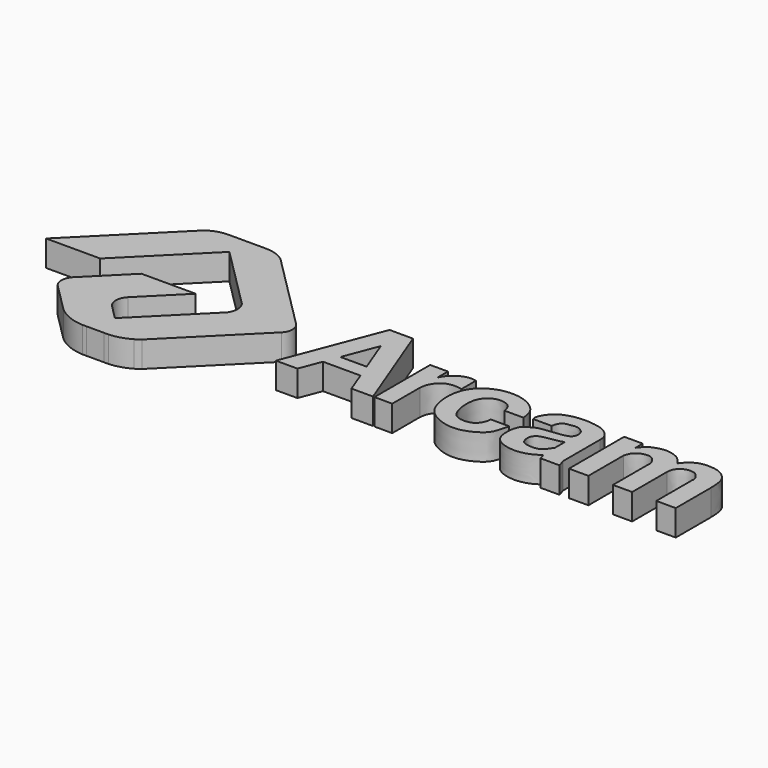
from build123d import *

# Parameters (mm, degrees)
F1_DEPTH = 2


# Not quite as in the source:
# - ends of sketch curves that miss each other by under 0.0002 mm in the source are joined


with BuildPart() as f1:
    # F0 (on Top) → F1 (new body)
    with BuildSketch(Plane.XY):
        with BuildLine():
            Line((-68.5442758233, 37.8376201657), (-75.2842758233, 31.0976201657))
            Line((-75.2842758233, 31.0976201657), (-71.1123458143, 31.0976201657))
            Line((-71.1123458143, 31.0976201657), (-65.5848875755, 36.6250784045))
            Line((-65.5848875755, 36.6250784045), (-64.6773347005, 37.5326312795))
            ThreePointArc((-64.6773347005, 37.5326312795), (-63.7017726464, 38.0238729513), (-62.6255051316, 37.8376259696))
            ThreePointArc((-62.6255051316, 37.8376259696), (-63.3349333998, 38.2093307968), (-64.1254993276, 38.3376213265))
            Line((-64.1254993276, 38.3376213265), (-67.0442758233, 38.3376201657))
            ThreePointArc((-67.0442758233, 38.3376201657), (-67.8348452384, 38.2093284108), (-68.5442758233, 37.8376201657))
        make_face()
        with BuildLine():
            Line((-64.6773347005, 37.5326312795), (-65.5848875755, 36.6250784045))
            Line((-65.5848875755, 36.6250784045), (-60.7645361178, 31.8047269468))
            ThreePointArc((-60.7645361178, 31.8047269468), (-60.5380345874, 31.0976201657), (-60.7645361178, 30.3905133845))
            Line((-60.7645361178, 30.3905133845), (-65.5722546007, 25.5827949015))
            Line((-65.5722546007, 25.5827949015), (-64.4237848444, 24.4343251452))
            ThreePointArc((-64.4237848444, 24.4343251452), (-63.7272467457, 24.0680817951), (-62.9458155435, 24.161166653))
            ThreePointArc((-62.9458155435, 24.161166653), (-62.7347896268, 24.2795555552), (-62.5487943481, 24.4343251452))
            Line((-62.5487943481, 24.4343251452), (-56.5926061088, 30.3905133845))
            ThreePointArc((-56.5926061088, 30.3905133845), (-56.29971289, 31.0976201657), (-56.5926061088, 31.8047269468))
            Line((-56.5926061088, 31.8047269468), (-62.6255051316, 37.8376259696))
            ThreePointArc((-62.6255051316, 37.8376259696), (-63.7017726464, 38.0238729513), (-64.6773347005, 37.5326312795))
        make_face()
        with BuildLine():
            Line((-64.4237848444, 24.4343251452), (-65.5722546007, 25.5827949015))
            Line((-65.5722546007, 25.5827949015), (-66.6552237276, 26.6657640284))
            ThreePointArc((-66.6552237276, 26.6657640284), (-66.9745179706, 27.4366085204), (-66.6552237276, 28.2074530124))
            Line((-66.6552237276, 28.2074530124), (-63.7650565743, 31.0976201657))
            Line((-63.7650565743, 31.0976201657), (-67.9369865833, 31.0976201657))
            Line((-67.9369865833, 31.0976201657), (-70.9051354279, 28.1294713211))
            ThreePointArc((-70.9051354279, 28.1294713211), (-71.1618860391, 27.4698706738), (-70.9545111372, 26.793121429))
            Line((-70.9545111372, 26.793121429), (-68.7112460172, 24.549856309))
            ThreePointArc((-68.7112460172, 24.549856309), (-67.7067925748, 23.9297700279), (-66.5533270991, 23.6788694294))
            Line((-66.5533270991, 23.6788694294), (-66.2402591376, 23.6788694294))
            Line((-66.2402591376, 23.6788694294), (-64.9042500639, 23.6788694294))
            Line((-64.9042500639, 23.6788694294), (-64.5486833954, 23.6788694294))
            ThreePointArc((-64.5486833954, 23.6788694294), (-63.7179930832, 23.8227872907), (-62.9458155435, 24.161166653))
            ThreePointArc((-62.9458155435, 24.161166653), (-63.7272467457, 24.0680817951), (-64.4237848444, 24.4343251452))
        make_face()
        with BuildLine():
            ThreePointArc((-64.9042500639, 23.6788694294), (-64.7264667296, 23.6743512397), (-64.5486833954, 23.6788694294))
            Line((-64.5486833954, 23.6788694294), (-64.9042500639, 23.6788694294))
        make_face()
        with BuildLine():
            ThreePointArc((-66.5533270991, 23.6788694294), (-66.3967931184, 23.6753672648), (-66.2402591376, 23.6788694294))
            Line((-66.2402591376, 23.6788694294), (-66.5533270991, 23.6788694294))
        make_face()
    extrude(amount=F1_DEPTH)


with BuildPart() as f1b:
    # F0 (on Top) → F1, piece 2 (new body)
    with BuildSketch(Plane.XY):
        Polygon((-51.7120547432, 34.7021047027), (-54.5506963793, 27.307190418), (-52.8916748268, 27.307190418), (-52.2540972099, 28.9681368956), (-49.3647159226, 28.9681368956), (-48.7271383057, 27.307190418), (-47.0681167532, 27.307190418), (-49.9067583893, 34.7021047027), align=None)
        Polygon((-49.8006260827, 30.103721687), (-51.8181870498, 30.103721687), (-50.8094065663, 32.7316846933), align=None, mode=Mode.SUBTRACT)
    extrude(amount=F1_DEPTH)


with BuildPart() as f1c:
    # F0 (on Top) → F1, piece 3 (new body)
    with BuildSketch(Plane.XY):
        with BuildLine():
            Line((-46.9542004939, 32.6685147129), (-46.9542004939, 27.3020714057))
            Line((-46.9542004939, 27.3020714057), (-45.5843665477, 27.3020714057))
            Line((-45.5843665477, 27.3020714057), (-45.5843665477, 29.9733391266))
            add(Edge.make_bspline(
                [(-43.5228206988, 31.4098937788), (-43.7790188564, 31.4438715653), (-44.2889116925, 31.5114951193), (-45.0377190249, 31.2578918185), (-45.509767693, 30.5488637582), (-45.5609753311, 30.153800628), (-45.5843665477, 29.9733391266)],
                knots=[0, 0, 0, 0, 0.257839139, 0.513158764, 0.777615035, 1, 1, 1, 1], degree=3))
            Line((-43.5228206988, 31.4098937788), (-43.5228206988, 32.7752627899))
            add(Edge.make_bspline(
                [(-45.5843665477, 31.6332013581), (-45.5308791384, 31.7621508466), (-45.4091654003, 32.0555829737), (-44.8749149339, 32.5566936661), (-44.3047762851, 32.8102137143), (-43.8681395106, 32.8598250997), (-43.634032553, 32.8024965546), (-43.5228206988, 32.7752627899)],
                knots=[0, 0, 0, 0, 0.1877342824, 0.4272003744, 0.6508029702, 0.8341149295, 1, 1, 1, 1], degree=3))
            Line((-45.5843665477, 31.6332013581), (-45.5843665477, 32.6685147129))
            Line((-45.5843665477, 32.6685147129), (-46.9542004939, 32.6685147129))
        make_face()
    extrude(amount=F1_DEPTH)


with BuildPart() as f1d:
    # F0 (on Top) → F1, piece 4 (new body)
    with BuildSketch(Plane.XY):
        with BuildLine():
            add(Edge.make_bspline(
                [(-39.6801316019, 29.3991039043), (-39.686803112, 29.285606014), (-39.7025314604, 29.0180302584), (-40.0586952504, 28.3565075453), (-40.8758640399, 28.2171193732), (-41.6480504786, 28.3931997992), (-42.0295799075, 29.2424037891), (-42.1067274766, 30.0710754063), (-42.0134657598, 30.937322568), (-41.4926872917, 31.5521784316), (-40.8688924084, 31.7306931298), (-40.4783101538, 31.6987941016), (-39.9004155078, 31.489165708), (-39.7861510004, 31.0446192871), (-39.7259787496, 30.8105189588)],
                knots=[0, 0, 0, 0, 0.0622431539, 0.1467406917, 0.2371908674, 0.3244821331, 0.4187817737, 0.5131626165, 0.6072061478, 0.6967160217, 0.7765125725, 0.8405526314, 0.9160342327, 1, 1, 1, 1], degree=3))
            Line((-39.7259787496, 30.8105189588), (-38.2851146933, 30.8105189588))
            add(Edge.make_bspline(
                [(-38.2851146933, 30.8105189588), (-38.3129706614, 31.1006446346), (-38.3732513436, 31.7284804208), (-39.3000192438, 32.6158305226), (-40.7352235549, 32.9369331543), (-42.0807149642, 32.6661135747), (-43.1941550306, 31.8261832119), (-43.6243075168, 30.6094778009), (-43.5687919539, 29.1385505177), (-42.9938653151, 27.8851633248), (-41.6243843874, 27.1631561296), (-40.1884811147, 27.0655135577), (-38.7419079117, 27.8532413643), (-38.4498668919, 28.5743798747), (-38.3214114992, 29.1184334886), (-38.2552341398, 29.3991039043)],
                knots=[0, 0, 0, 0, 0.0649865704, 0.1406361539, 0.2238339965, 0.3043934108, 0.3839580048, 0.4612270243, 0.5445450075, 0.6241267959, 0.7077336197, 0.7910379039, 0.8768844905, 0.9365324786, 1, 1, 1, 1], degree=3))
            Line((-38.2552341398, 29.3991039043), (-39.6801316019, 29.3991039043))
        make_face()
    extrude(amount=F1_DEPTH)


with BuildPart() as f1e:
    # F0 (on Top) → F1, piece 5 (new body)
    with BuildSketch(Plane.XY):
        with BuildLine():
            Line((-37.7291685499, 31.0345437839), (-36.2866274836, 31.0345437839))
            add(Edge.make_bspline(
                [(-36.2866274836, 31.0345437839), (-36.2639665838, 31.1632808649), (-36.2180610598, 31.4216417454), (-35.9418161151, 31.7712931723), (-35.4547206246, 31.8210455176), (-34.8890495017, 31.9372236855), (-34.2592396767, 31.463515402), (-34.3472953032, 30.8675106063), (-34.6514716049, 30.502926623), (-36.323384653, 30.4173959993), (-36.9633353247, 30.2446408368), (-37.3439883665, 29.9664238094), (-37.7053006369, 29.8256006934), (-37.9324217031, 29.040710271), (-37.8966421526, 28.4631068949), (-37.8236406423, 27.9595767044), (-37.3675917674, 27.3718102767), (-36.1089928004, 27.0435627252), (-34.9973249818, 27.2984230003), (-34.5218174602, 27.6168176867), (-34.3029709138, 27.7626998882)],
                knots=[0, 0, 0, 0, 0.0430832367, 0.0868159876, 0.1339912459, 0.1859479856, 0.2428756159, 0.2922117824, 0.3369134525, 0.4249221782, 0.4829217533, 0.5279091842, 0.5691418842, 0.6293262067, 0.6827371289, 0.730345257, 0.7872122129, 0.8645836121, 0.9378736204, 1, 1, 1, 1], degree=3))
            Line((-34.3029709138, 27.7626998882), (-34.1903889157, 27.316307665))
            Line((-34.1903889157, 27.316307665), (-32.7000120259, 27.316307665))
            Line((-32.7000120259, 27.316307665), (-32.8900722558, 27.8605339277))
            Line((-32.8900722558, 27.8605339277), (-32.8900722558, 31.4506291681))
            add(Edge.make_bspline(
                [(-37.7291685499, 31.0345437839), (-37.7470281811, 31.1266932346), (-37.7912274188, 31.3545349412), (-37.4767345128, 31.9664452879), (-36.9299903055, 32.4866545208), (-36.1125854833, 32.8104359702), (-35.0252060713, 32.8892615099), (-34.2833706877, 32.7878660836), (-33.4811828772, 32.6042775712), (-32.8771034922, 31.9162214757), (-32.8900722558, 31.5882499932), (-32.8900722558, 31.4506291681)],
                knots=[0, 0, 0, 0, 0.0726925151, 0.1796667687, 0.2947703493, 0.4185956983, 0.5562149551, 0.6714091926, 0.790672085, 0.9125878862, 1, 1, 1, 1], degree=3))
        make_face()
        with BuildLine():
            add(Edge.make_bspline(
                [(-34.3537897643, 29.922141413), (-34.4036580061, 29.8817344179), (-34.5568041392, 29.7634813159), (-35.457999965, 29.6337546115), (-36.0833828843, 29.5439273316), (-36.4431169809, 29.1679387323), (-36.4507740138, 28.7551650582), (-36.3332154987, 28.3862247952), (-36.0471524731, 28.1579445459), (-34.9480402798, 28.0901852172), (-34.6182196791, 28.5401996718), (-34.4420837444, 28.8040190114), (-34.3537897643, 28.9315419054)],
                knots=[0, 0, 0, 0, 0.0673991169, 0.2001580081, 0.3140693774, 0.4084334618, 0.4963213211, 0.580116407, 0.6625144488, 0.8036967744, 0.9045160286, 1, 1, 1, 1], degree=3))
            Line((-34.3537897643, 29.922141413), (-34.3537897643, 28.9315419054))
        make_face(mode=Mode.SUBTRACT)
    extrude(amount=F1_DEPTH)


with BuildPart() as f1f:
    # F0 (on Top) → F1, piece 6 (new body)
    with BuildSketch(Plane.XY):
        with BuildLine():
            Line((-30.4993697282, 27.3333645427), (-30.4993697282, 30.7066261421))
            add(Edge.make_bspline(
                [(-28.6074102696, 30.7066261421), (-28.5956726296, 30.7942236475), (-28.5690850817, 30.9926453809), (-28.8068489541, 31.3843936808), (-29.1174767373, 31.683481058), (-29.7283563502, 31.6363493313), (-30.1075932086, 31.4416108404), (-30.3919188743, 31.1127021721), (-30.4634839564, 30.8422449037), (-30.4993697282, 30.7066261421)],
                knots=[0, 0, 0, 0, 0.1156086525, 0.261871261, 0.4040802558, 0.5706661941, 0.715425248, 0.8573021325, 1, 1, 1, 1], degree=3))
            Line((-28.6074102696, 30.7066261421), (-28.6074102696, 27.3333645427))
            Line((-28.6074102696, 27.3333645427), (-27.126287001, 27.3333645427))
            Line((-27.126287001, 27.3333645427), (-27.126287001, 30.7066261421))
            add(Edge.make_bspline(
                [(-25.2696805473, 30.7066261421), (-25.2553864617, 30.8161199086), (-25.2251709647, 31.047572878), (-25.4717717253, 31.4049990867), (-25.773658954, 31.7011130248), (-26.4883715447, 31.6956734186), (-26.877713314, 31.3712772603), (-27.0782341365, 31.0962156803), (-27.1098185492, 30.8401444373), (-27.126287001, 30.7066261421)],
                knots=[0, 0, 0, 0, 0.1258615218, 0.2660518846, 0.4065038542, 0.584818524, 0.7387613839, 0.863787381, 1, 1, 1, 1], degree=3))
            Line((-25.2696805473, 30.7066261421), (-25.2696805473, 27.3333645427))
            Line((-25.2696805473, 27.3333645427), (-23.7707112756, 27.3333645427))
            Line((-23.7707112756, 27.3333645427), (-23.7707112756, 30.7066261421))
            add(Edge.make_bspline(
                [(-27.3285423245, 31.9559838508), (-27.234633537, 32.0788311225), (-27.0262591138, 32.3514172145), (-26.4153201488, 32.8028650006), (-25.6285680976, 32.8757245453), (-24.7521374327, 32.780029561), (-24.0948733512, 32.2581251103), (-23.8133343477, 31.7150296498), (-23.7861526351, 31.0719475595), (-23.7707112756, 30.7066261421)],
                knots=[0, 0, 0, 0, 0.1160288221, 0.2574566186, 0.4042732369, 0.5591955289, 0.7065864858, 0.8333179503, 1, 1, 1, 1], degree=3))
            add(Edge.make_bspline(
                [(-30.5705712017, 31.9559838508), (-30.5159518597, 32.0277110652), (-30.3896717682, 32.1935446118), (-30.0581701082, 32.5681032795), (-29.13838503, 32.8753772603), (-28.4916604671, 32.8083701255), (-27.8302641592, 32.593462596), (-27.5014849849, 32.1757216866), (-27.3285423245, 31.9559838508)],
                knots=[0, 0, 0, 0, 0.1128845328, 0.2609893971, 0.466819193, 0.6388453034, 0.8100273407, 1, 1, 1, 1], degree=3))
            Line((-30.5705712017, 31.9559838508), (-30.5705712017, 32.6522020159))
            Line((-30.5705712017, 32.6522020159), (-31.9990039643, 32.6522020159))
            Line((-31.9990039643, 32.6522020159), (-31.9990039643, 27.3333645427))
            Line((-31.9990039643, 27.3333645427), (-30.4993697282, 27.3333645427))
        make_face()
    extrude(amount=F1_DEPTH)


solid = Compound([f1.part, f1b.part, f1c.part, f1d.part, f1e.part, f1f.part])
